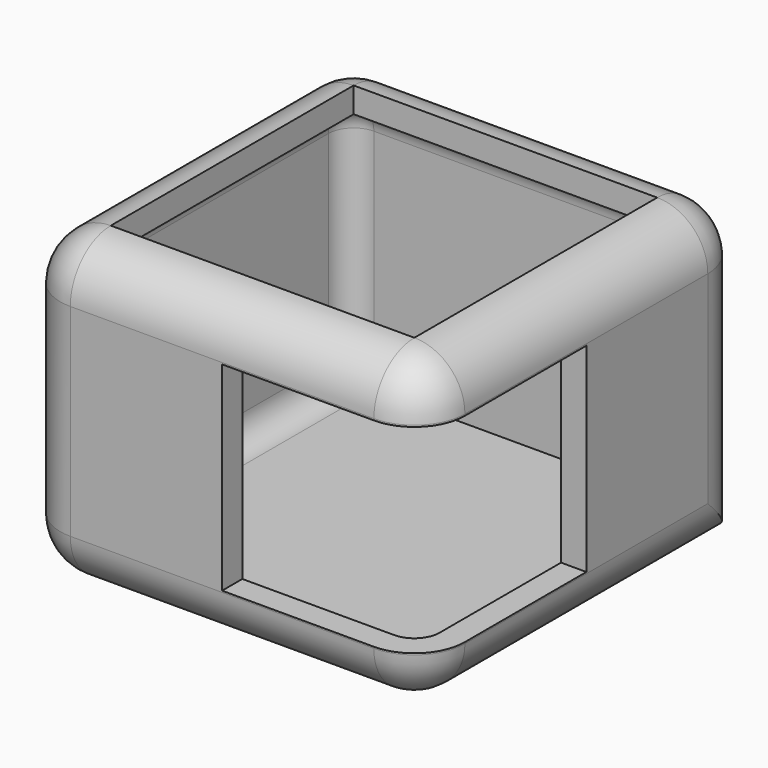
from build123d import *

# Parameters (mm, degrees)
F0_W     = 40
F0_H     = 40
F1_DEPTH = 30
F2_R     = 5
F3_T     = -2.5
F4_W     = 20.2598124743
F4_H     = 19.6875007823
F5_DEPTH = 61


# Not quite as in the source:
# - a shell that OpenCascade refuses in one call is made with other operations: the cavity is built on its own and cut out


with BuildPart() as f1:
    # F0 (on Top) → F1 (new body)
    with BuildSketch(Plane.XY):
        Rectangle(F0_W, F0_H)
    extrude(amount=F1_DEPTH)

    # F2
    f2_edges = [f1.edges().sort_by_distance(p)[0] for p in [
        (-20, -20, 15),
        (20, -20, 15),
        (0, -20, 0),
        (0, -20, 30),
        (-20, 0, 30),
        (20, 0, 30),
        (0, 20, 30),
        (20, 20, 15),
        (20, 0, 0),
        (-20, 20, 15),
        (-20, 0, 0),
    ]]
    fillet(f2_edges, radius=F2_R)

    # F3: a shell. OpenCascade refuses it in one call, so the cavity is built on its own and cut out:
    # the body offset inwards by the wall thickness, plus a prism from it out through each open face.
    f3_core = offset(f1.part, amount=F3_T, mode=Mode.PRIVATE)
    f3_exits = [f3_core.faces().sort_by_distance(p)[0] for p in [
        (0, 0, 27.5),
    ]]
    add(f3_core, mode=Mode.SUBTRACT)
    extrude(f3_exits, amount=-F3_T, mode=Mode.SUBTRACT)

    # F4 (on Front) → F5 (cut)
    with BuildSketch(Plane.XZ):
        with Locations((10.1299062371, 14.9945500307)):
            Rectangle(F4_W, F4_H)
    extrude(amount=F5_DEPTH, mode=Mode.SUBTRACT)


solid = f1.part
